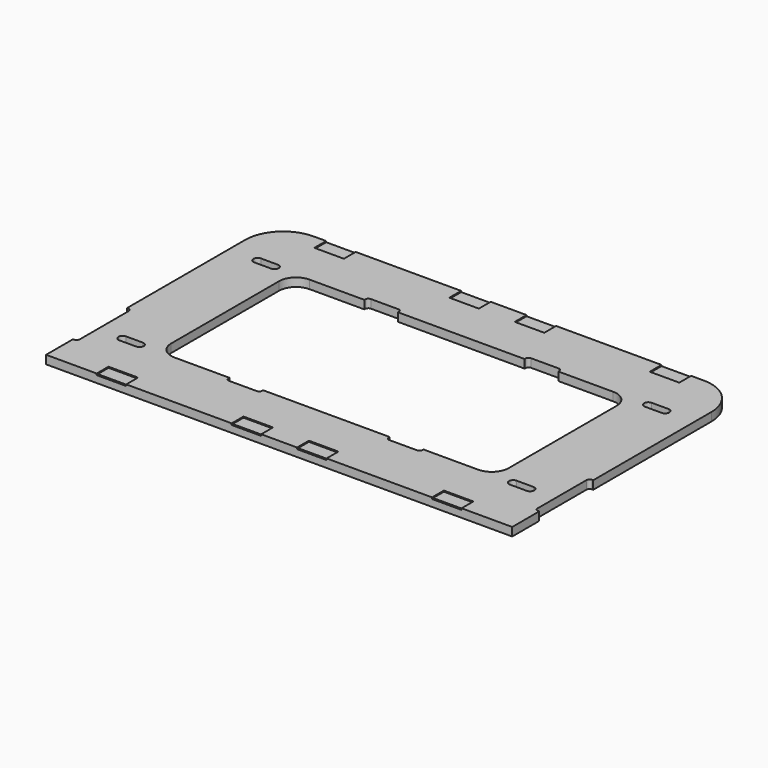
from build123d import *

# Parameters (mm, degrees)
F0_W      = 1403.35
F0_H      = 863.6
F1_DEPTH  = 25.4
F3_DEPTH  = 25.4
F4_W      = 88.9
F4_H      = 44.45
F5_DEPTH  = 3.175
F6_W      = 88.9
F6_H      = 3.81
F7_DEPTH  = 4.445
F8_R      = 114.3
F9_W      = 88.9
F9_H      = 44.45
F10_DEPTH = 3.175
F11_W     = 12.7
F11_H     = 203.2
F12_DEPTH = 25.401
F13_R     = 9.525
F14_W     = 101.6
F14_H     = 12.7
F15_DEPTH = 25.401
F16_R     = 9.525
F17_W     = 76.2
F17_H     = 25.4
F18_DEPTH = 25.401
F19_R     = 12.69999


# Not quite as in the source:
# - a fillet or chamfer is up to 0.001 mm smaller than in the source, because OpenCascade refuses the exact size


with BuildPart() as f1:
    # F0 (on Top) → F1 (new body)
    with BuildSketch(Plane.XY):
        Rectangle(F0_W, F0_H)
    extrude(amount=F1_DEPTH)

    # F2 (on face) → F3 (cut)
    with BuildSketch(Plane.XY.offset(25.4)):
        with BuildLine():
            Line((457.2, 254), (-457.2, 254))
            ThreePointArc((-457.2, 254), (-493.1210244843, 239.1210244843), (-508, 203.2))
            Line((-508, 203.2), (-508, -203.2))
            ThreePointArc((-508, -203.2), (-493.1210244843, -239.1210244843), (-457.2, -254))
            Line((-457.2, -254), (457.2, -254))
            ThreePointArc((457.2, -254), (493.1210244843, -239.1210244843), (508, -203.2))
            Line((508, -203.2), (508, 203.2))
            ThreePointArc((508, 203.2), (493.1210244843, 239.1210244843), (457.2, 254))
        make_face()
    extrude(amount=-F3_DEPTH, mode=Mode.SUBTRACT)

    # F4 (on face) → F5 (cut)
    with BuildSketch(Plane.XY.offset(25.4)):
        with Locations((-504.825, -409.575)):
            Rectangle(F4_W, F4_H)
        with Locations((-98.425, -409.575)):
            Rectangle(F4_W, F4_H)
        with Locations((98.425, -409.575)):
            Rectangle(F4_W, F4_H)
        with Locations((504.825, -409.575)):
            Rectangle(F4_W, F4_H)
    extrude(amount=-F5_DEPTH, mode=Mode.SUBTRACT)

    # F6 (on face) → F7 (cut)
    with BuildSketch(Plane.XY.offset(25.4)):
        with Locations((-504.825, -429.895)):
            Rectangle(F6_W, F6_H)
        with Locations((-98.425, -429.895)):
            Rectangle(F6_W, F6_H)
        with Locations((98.425, -429.895)):
            Rectangle(F6_W, F6_H)
        with Locations((504.825, -429.895)):
            Rectangle(F6_W, F6_H)
    extrude(amount=-F7_DEPTH, mode=Mode.SUBTRACT)

    # F8
    f8_edges = [f1.edges().sort_by_distance(p)[0] for p in [
        (701.675, 431.8, 12.7),
        (-701.675, 431.8, 12.7),
    ]]
    fillet(f8_edges, radius=F8_R)

    # F9 (on face) → F10 (cut)
    with BuildSketch(Plane.XY.offset(25.4)):
        with Locations((98.425, 409.575)):
            Rectangle(F9_W, F9_H)
        with Locations((504.825, 409.575)):
            Rectangle(F9_W, F9_H)
        with Locations((-98.425, 409.575)):
            Rectangle(F9_W, F9_H)
        with Locations((-504.825, 409.575)):
            Rectangle(F9_W, F9_H)
    extrude(amount=-F10_DEPTH, mode=Mode.SUBTRACT)

    # F11 (on face) → F12 (cut, through all)
    with BuildSketch(Plane.XY.offset(25.4)):
        with Locations((-695.325, -228.6)):
            Rectangle(F11_W, F11_H)
        with Locations((695.325, -228.6)):
            Rectangle(F11_W, F11_H)
    extrude(amount=-F12_DEPTH, mode=Mode.SUBTRACT)

    # F13
    f13_edges = [f1.edges().sort_by_distance(p)[0] for p in [
        (-688.975, -127, 12.7),
        (-688.975, -330.2, 12.7),
        (688.975, -127, 12.7),
        (688.975, -330.2, 12.7),
    ]]
    fillet(f13_edges, radius=F13_R)

    # F14 (on face) → F15 (cut, through all)
    with BuildSketch(Plane.XY.offset(25.4)):
        with Locations((-241.3, -260.35)):
            Rectangle(F14_W, F14_H)
        with Locations((241.3, -260.35)):
            Rectangle(F14_W, F14_H)
        with Locations((-241.3, 260.35)):
            Rectangle(F14_W, F14_H)
        with Locations((241.3, 260.35)):
            Rectangle(F14_W, F14_H)
    extrude(amount=-F15_DEPTH, mode=Mode.SUBTRACT)

    # F16
    f16_edges = [f1.edges().sort_by_distance(p)[0] for p in [
        (-292.1, -266.7, 12.7),
        (190.5, -266.7, 12.7),
        (292.1, -266.7, 12.7),
        (-190.5, -266.7, 12.7),
        (190.5, 266.7, 12.7),
        (-292.1, 266.7, 12.7),
        (-190.5, 266.7, 12.7),
        (292.1, 266.7, 12.7),
    ]]
    fillet(f16_edges, radius=F16_R)

    # F17 (on face) → F18 (cut, through all)
    with BuildSketch(Plane.XY.offset(25.4)):
        with Locations((-588.01, 254)):
            Rectangle(F17_W, F17_H)
        with Locations((588.01, 254)):
            Rectangle(F17_W, F17_H)
        with Locations((588.01, -254)):
            Rectangle(F17_W, F17_H)
        with Locations((-588.01, -254)):
            Rectangle(F17_W, F17_H)
    extrude(amount=-F18_DEPTH, mode=Mode.SUBTRACT)

    # F19 (radius 12.7 in the source; OpenCascade refuses exactly that, so slightly less here)
    f19_edges = [f1.edges().sort_by_distance(p)[0] for p in [
        (-626.11, 241.3, 12.7),
        (-549.91, 241.3, 12.7),
        (-549.91, 266.7, 12.7),
        (-626.11, 266.7, 12.7),
        (-626.11, -241.3, 12.7),
        (-626.11, -266.7, 12.7),
        (-549.91, -266.7, 12.7),
        (-549.91, -241.3, 12.7),
        (626.11, -241.3, 12.7),
        (626.11, -266.7, 12.7),
        (549.91, -266.7, 12.7),
        (549.91, -241.3, 12.7),
        (549.91, 266.7, 12.7),
        (549.91, 241.3, 12.7),
        (626.11, 241.3, 12.7),
        (626.11, 266.7, 12.7),
    ]]
    fillet(f19_edges, radius=F19_R)


solid = f1.part
